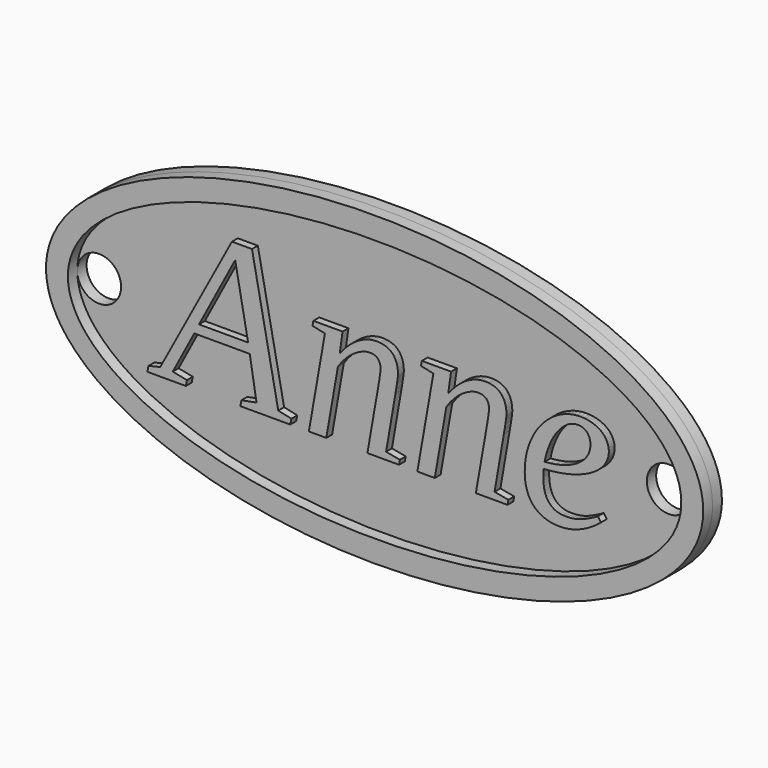
from build123d import *

# Parameters (mm, degrees)
F0_R     = 3
F1_DEPTH = 1.6
F2_DEPTH = 1.6
F3_DEPTH = 1


with BuildPart() as f1:
    # F0 (on Front) → F1 (new body)
    with BuildSketch(Plane.XZ):
        with BuildLine():
            add(Edge.make_bspline(
                [(45, 0), (45, 36.3730669589), (-22.5, 18.1865334795), (-90, 0), (-22.5, -18.1865334795), (45, -36.3730669589), (45, 0)],
                knots=[0, 0, 0, 2.0943951024, 2.0943951024, 4.1887902048, 4.1887902048, 6.2831853072, 6.2831853072, 6.2831853072], degree=2, weights=[1, 0.5, 1, 0.5, 1, 0.5, 1]))
        make_face()
        with BuildLine():
            add(Edge.make_bspline(
                [(42, 0), (42, 17.9999999333), (1.556e-07, 18), (-41.9999996887, 18.0000000667), (-42, 1.334e-07)],
                knots=[0, 0, 0, 1.5707963231, 1.5707963231, 3.1415926462, 3.1415926462, 3.1415926462], degree=2, weights=[1, 0.7071067825, 1, 0.7071067825, 1]))
            add(Edge.make_bspline(
                [(-42, 1.334e-07), (-42.0000003113, -17.9999999333), (-1.556e-07, -18), (42, -18.0000000667), (42, 0)],
                knots=[3.1415926462, 3.1415926462, 3.1415926462, 4.7123889767, 4.7123889767, 6.2831853072, 6.2831853072, 6.2831853072], degree=2, weights=[1, 0.7071067799, 1, 0.7071067799, 1]))
        make_face(mode=Mode.SUBTRACT)
        with BuildLine():
            add(Edge.make_bspline(
                [(-42, 1.334e-07), (-42.0000003113, -17.9999999333), (-1.556e-07, -18), (42, -18.0000000667), (42, 0)],
                knots=[3.1415926462, 3.1415926462, 3.1415926462, 4.7123889767, 4.7123889767, 6.2831853072, 6.2831853072, 6.2831853072], degree=2, weights=[1, 0.7071067799, 1, 0.7071067799, 1]))
            add(Edge.make_bspline(
                [(42, 0), (42, 17.9999999333), (1.556e-07, 18), (-41.9999996887, 18.0000000667), (-42, 1.334e-07)],
                knots=[0, 0, 0, 1.5707963231, 1.5707963231, 3.1415926462, 3.1415926462, 3.1415926462], degree=2, weights=[1, 0.7071067825, 1, 0.7071067825, 1]))
        make_face()
        Polygon((0.3302, 2.3205647869), (0.3306, 2.3652647869), (0.3252, 2.5233647869), (0.3185, 2.5995647869), (0.3091, 2.6737647869), (0.2969, 2.7461647869), (0.2821, 2.8165647869), (0.2645, 2.8851647869), (0.2443, 2.9517647869), (0.2214, 3.0164647869), (0.1957, 3.0792647869), (0.1674, 3.1401647869), (0.1363, 3.1991647869), (0.1026, 3.2561647869), (0.0662, 3.3113647869), (0.0271, 3.3645647869), (-0.0148, 3.4158647869), (-0.0595, 3.4646647869), (-0.1074, 3.5103647869), (-0.1585, 3.5528647869), (-0.2127, 3.5921647869), (-0.27, 3.6283647869), (-0.3305, 3.6614647869), (-0.3941, 3.6913647869), (-0.4609, 3.7181647869), (-0.5309, 3.7417647869), (-0.6039, 3.7621647869), (-0.6802, 3.7795647869), (-0.7596, 3.7936647869), (-0.8421, 3.8046647869), (-0.9278, 3.8125647869), (-1.0166, 3.8172647869), (-1.1086, 3.8188647869), (-1.2601, 3.8143647869), (-1.4126, 3.8008647869), (-1.566, 3.7783647869), (-1.7202, 3.7469647869), (-1.8754, 3.7064647869), (-2.0315, 3.6569647869), (-2.1884, 3.5984647869), (-2.3463, 3.5310647869), (-2.6602, 3.3835647869), (-2.9688, 3.2143647869), (-3.2719, 3.0237647869), (-3.5696, 2.8114647869), (-3.8593, 2.5802647869), (-4.1381, 2.3328647869), (-4.4062, 2.0693647869), (-4.6634, 1.7895647869), (-4.9054, 1.5089647869), (-5.1276, 1.2282647869), (-5.33, 0.9476647869), (-5.5126, 0.6669647869), (-7.0957, -8.4000352131), (-9.4848, -8.4000352131), (-7.2828, 4.1354647869), (-8.9811, 4.4952647869), (-8.8659, 5.1429647869), (-4.8649, 5.1429647869), (-5.2535, 2.3796647869), (-4.9774, 2.7241647869), (-4.4089, 3.3646647869), (-4.1165, 3.6605647869), (-3.8125, 3.9376647869), (-3.5049, 4.1930647869), (-3.1936, 4.4269647869), (-2.8788, 4.6392647869), (-2.5541, 4.8290647869), (-2.2276, 4.9954647869), (-1.8992, 5.1384647869), (-1.5691, 5.2580647869), (-1.23, 5.3588647869), (-0.8891, 5.4307647869), (-0.5464, 5.4739647869), (-0.2019, 5.4883647869), (0.1211, 5.4775647869), (0.2764, 5.4640647869), (0.4278, 5.4451647869), (0.5751, 5.4208647869), (0.7183, 5.3912647869), (0.8575, 5.3561647869), (0.9927, 5.3156647869), (1.1267, 5.2693647869), (1.2553, 5.2167647869), (1.3786, 5.1577647869), (1.4964, 5.0925647869), (1.6088, 5.0210647869), (1.7159, 4.9432647869), (1.8175, 4.8591647869), (1.9138, 4.7687647869), (2.008, 4.6720647869), (2.0964, 4.5690647869), (2.1789, 4.4597647869), (2.2556, 4.3441647869), (2.3264, 4.2222647869), (2.3914, 4.0941647869), (2.4506, 3.9596647869), (2.5039, 3.8188647869), (2.5545, 3.6715647869), (2.5983, 3.5175647869), (2.6354, 3.3567647869), (2.6658, 3.1892647869), (2.6894, 3.0149647869), (2.7062, 2.8339647869), (2.7164, 2.6461647869), (2.7197, 2.4516647869), (2.7196, 2.4295647869), (2.7191, 2.4064647869), (2.717, 2.3571647869), (2.7137, 2.3038647869), (2.7089, 2.2465647869), (2.7029, 2.1851647869), (2.6954, 2.1196647869), (2.6867, 2.0502647869), (2.6766, 1.9766647869), (2.6604, 1.8291647869), (2.6406, 1.6744647869), (2.6172, 1.5125647869), (2.5902, 1.3434647869), (2.5614, 1.1689647869), (2.5039, 0.8091647869), (2.4751, 0.6238647869), (2.4463, 0.4466647869), (2.3887, 0.1083647869), (2.3599, -0.0526352131), (1.0934, -7.4069352131), (2.9788, -7.7524352131), (2.8637, -8.4000352131), (-1.4684, -8.4000352131), (-0.0004, -0.0238352131), (0.0284, 0.1362647869), (0.086, 0.4673647869), (0.1148, 0.6382647869), (0.1426, 0.8100647869), (0.193, 1.1482647869), (0.2155, 1.3146647869), (0.2425, 1.4765647869), (0.2659, 1.6312647869), (0.2857, 1.7787647869), (0.3019, 1.9191647869), (0.3086, 1.9858647869), (0.3145, 2.0495647869), (0.3194, 2.1100647869), (0.3234, 2.1673647869), (0.3266, 2.2215647869), (0.3288, 2.2726647869), align=None, mode=Mode.SUBTRACT)
        Polygon((15.1836, 2.3205647869), (15.184, 2.3652647869), (15.1786, 2.5233647869), (15.1719, 2.5995647869), (15.1624, 2.6737647869), (15.1503, 2.7461647869), (15.1355, 2.8165647869), (15.1179, 2.8851647869), (15.0977, 2.9517647869), (15.0747, 3.0164647869), (15.0491, 3.0792647869), (15.0208, 3.1401647869), (14.9897, 3.1991647869), (14.956, 3.2561647869), (14.9196, 3.3113647869), (14.8805, 3.3645647869), (14.8386, 3.4158647869), (14.7939, 3.4646647869), (14.746, 3.5103647869), (14.6949, 3.5528647869), (14.6407, 3.5921647869), (14.5834, 3.6283647869), (14.5229, 3.6614647869), (14.4593, 3.6913647869), (14.3925, 3.7181647869), (14.3225, 3.7417647869), (14.2494, 3.7621647869), (14.1732, 3.7795647869), (14.0938, 3.7936647869), (14.0113, 3.8046647869), (13.9256, 3.8125647869), (13.8368, 3.8172647869), (13.7448, 3.8188647869), (13.5933, 3.8143647869), (13.4408, 3.8008647869), (13.2874, 3.7783647869), (13.1332, 3.7469647869), (12.978, 3.7064647869), (12.8219, 3.6569647869), (12.665, 3.5984647869), (12.5071, 3.5310647869), (12.1932, 3.3835647869), (11.8846, 3.2143647869), (11.5815, 3.0237647869), (11.2838, 2.8114647869), (10.9941, 2.5802647869), (10.7153, 2.3328647869), (10.4472, 2.0693647869), (10.19, 1.7895647869), (9.948, 1.5089647869), (9.7258, 1.2282647869), (9.5234, 0.9476647869), (9.3408, 0.6669647869), (7.7577, -8.4000352131), (5.3686, -8.4000352131), (7.5706, 4.1354647869), (5.8723, 4.4952647869), (5.9875, 5.1429647869), (9.9885, 5.1429647869), (9.5999, 2.3796647869), (9.876, 2.7241647869), (10.4445, 3.3646647869), (10.7369, 3.6605647869), (11.0409, 3.9376647869), (11.3485, 4.1930647869), (11.6598, 4.4269647869), (11.9746, 4.6392647869), (12.2993, 4.8290647869), (12.6258, 4.9954647869), (12.9542, 5.1384647869), (13.2843, 5.2580647869), (13.6234, 5.3588647869), (13.9643, 5.4307647869), (14.307, 5.4739647869), (14.6515, 5.4883647869), (14.9745, 5.4775647869), (15.1298, 5.4640647869), (15.2812, 5.4451647869), (15.4285, 5.4208647869), (15.5717, 5.3912647869), (15.7109, 5.3561647869), (15.8461, 5.3156647869), (15.9801, 5.2693647869), (16.1087, 5.2167647869), (16.232, 5.1577647869), (16.3498, 5.0925647869), (16.4622, 5.0210647869), (16.5693, 4.9432647869), (16.6709, 4.8591647869), (16.7672, 4.7687647869), (16.8614, 4.6720647869), (16.9498, 4.5690647869), (17.0323, 4.4597647869), (17.109, 4.3441647869), (17.1798, 4.2222647869), (17.2448, 4.0941647869), (17.304, 3.9596647869), (17.3572, 3.8188647869), (17.4078, 3.6715647869), (17.4517, 3.5175647869), (17.4888, 3.3567647869), (17.5192, 3.1892647869), (17.5428, 3.0149647869), (17.5596, 2.8339647869), (17.5698, 2.6461647869), (17.5731, 2.4516647869), (17.573, 2.4295647869), (17.5725, 2.4064647869), (17.5704, 2.3571647869), (17.5671, 2.3038647869), (17.5623, 2.2465647869), (17.5563, 2.1851647869), (17.5488, 2.1196647869), (17.5401, 2.0502647869), (17.53, 1.9766647869), (17.5138, 1.8291647869), (17.494, 1.6744647869), (17.4706, 1.5125647869), (17.4436, 1.3434647869), (17.4148, 1.1689647869), (17.3572, 0.8091647869), (17.3285, 0.6238647869), (17.2997, 0.4466647869), (17.2421, 0.1083647869), (17.2133, -0.0526352131), (15.9468, -7.4069352131), (17.8322, -7.7524352131), (17.7171, -8.4000352131), (13.385, -8.4000352131), (14.853, -0.0238352131), (14.8818, 0.1362647869), (14.9394, 0.4673647869), (14.9682, 0.6382647869), (14.996, 0.8100647869), (15.0464, 1.1482647869), (15.0689, 1.3146647869), (15.0959, 1.4765647869), (15.1193, 1.6312647869), (15.1391, 1.7787647869), (15.1553, 1.9191647869), (15.162, 1.9858647869), (15.1678, 2.0495647869), (15.1728, 2.1100647869), (15.1768, 2.1673647869), (15.18, 2.2215647869), (15.1822, 2.2726647869), align=None, mode=Mode.SUBTRACT)
        Polygon((31.5875, 2.6947647869), (31.5918, 2.5379647869), (31.5826, 2.3056647869), (31.5549, 2.0765647869), (31.5088, 1.8505647869), (31.4443, 1.6276647869), (31.3613, 1.4079647869), (31.2599, 1.1914647869), (31.14, 0.9779647869), (31.0017, 0.7677647869), (30.8456, 0.5615647869), (30.6725, 0.3602647869), (30.4822, 0.1639647869), (30.2749, -0.0274352131), (30.0505, -0.2138352131), (29.809, -0.3953352131), (29.5504, -0.5718352131), (29.2747, -0.7434352131), (28.9855, -0.9057352131), (28.6792, -1.0618352131), (28.3558, -1.2116352131), (28.0153, -1.3551352131), (27.6578, -1.4922352131), (27.2831, -1.6231352131), (26.4826, -1.8660352131), (25.6244, -2.0702352131), (24.7052, -2.2366352131), (23.7247, -2.3652352131), (22.6831, -2.4561352131), (22.6812, -2.4728352131), (22.6792, -2.4907352131), (22.6772, -2.5097352131), (22.675, -2.5298352131), (22.6727, -2.5511352131), (22.6702, -2.5734352131), (22.6677, -2.5969352131), (22.6651, -2.6216352131), (22.6594, -2.6742352131), (22.6534, -2.7313352131), (22.6469, -2.7929352131), (22.6399, -2.8590352131), (22.6365, -2.9290352131), (22.6311, -3.0783352131), (22.6275, -3.2402352131), (22.6257, -3.4147352131), (22.6255, -3.5067352131), (22.6336, -3.8566352131), (22.6579, -4.2011352131), (22.6983, -4.5402352131), (22.755, -4.8739352131), (22.7941, -5.0372352131), (22.8396, -5.1960352131), (22.8913, -5.3502352131), (22.9493, -5.5000352131), (23.0136, -5.6453352131), (23.0842, -5.7860352131), (23.1611, -5.9223352131), (23.2444, -6.0541352131), (23.3345, -6.1805352131), (23.4323, -6.3005352131), (23.5378, -6.4143352131), (23.6509, -6.5218352131), (23.7717, -6.6230352131), (23.9001, -6.7179352131), (24.0361, -6.8065352131), (24.1798, -6.8888352131), (24.3323, -6.9597352131), (24.4947, -7.0211352131), (24.6669, -7.0730352131), (24.8491, -7.1155352131), (25.0411, -7.1486352131), (25.2431, -7.1722352131), (25.4549, -7.1863352131), (25.6766, -7.1911352131), (25.9973, -7.1843352131), (26.3117, -7.1641352131), (26.6198, -7.1303352131), (26.9215, -7.0831352131), (27.217, -7.0224352131), (27.5062, -6.9482352131), (27.7891, -6.8605352131), (28.0657, -6.7593352131), (28.6036, -6.5290352131), (29.6255, -6.0253352131), (30.1094, -5.7518352131), (30.5268, -6.3563352131), (30.2866, -6.5524352131), (30.0266, -6.7521352131), (29.7469, -6.9554352131), (29.4474, -7.1623352131), (29.1307, -7.3665352131), (28.7997, -7.5617352131), (28.0945, -7.9251352131), (27.7293, -8.0834352131), (27.3533, -8.2273352131), (26.9665, -8.3568352131), (26.5689, -8.4720352131), (26.1642, -8.5664352131), (25.7558, -8.6339352131), (25.3438, -8.6743352131), (24.9282, -8.6878352131), (24.6273, -8.6824352131), (24.3364, -8.6663352131), (24.0553, -8.6393352131), (23.7841, -8.6015352131), (23.5227, -8.5529352131), (23.2713, -8.4935352131), (23.0298, -8.4234352131), (22.7982, -8.3424352131), (22.5762, -8.2480352131), (22.3637, -8.1445352131), (22.1607, -8.0321352131), (21.967, -7.9107352131), (21.7829, -7.7802352131), (21.6081, -7.6408352131), (21.4429, -7.4924352131), (21.287, -7.3350352131), (21.1406, -7.1686352131), (21.0037, -6.9932352131), (20.8762, -6.8088352131), (20.7581, -6.6154352131), (20.6495, -6.4130352131), (20.5503, -6.2016352131), (20.4606, -5.9812352131), (20.3803, -5.7518352131), (20.3095, -5.5144352131), (20.2481, -5.2697352131), (20.1961, -5.0179352131), (20.1536, -4.7588352131), (20.1206, -4.4925352131), (20.0828, -3.9384352131), (20.0781, -3.6506352131), (20.0961, -3.0173352131), (20.15, -2.3985352131), (20.24, -1.7940352131), (20.3659, -1.2039352131), (20.5242, -0.6247352131), (20.7113, -0.0670352131), (20.9272, 0.4690647869), (21.1719, 0.9836647869), (21.4435, 1.4819647869), (21.7404, 1.9550647869), (22.0624, 2.4030647869), (22.4096, 2.8258647869), (22.7766, 3.2278647869), (23.158, 3.5993647869), (23.5538, 3.9403647869), (23.964, 4.2506647869), (24.3939, 4.5285647869), (24.8347, 4.7723647869), (25.2862, 4.9819647869), (25.7486, 5.1573647869), (26.2253, 5.3021647869), (26.7057, 5.4055647869), (27.1896, 5.4676647869), (27.6771, 5.4883647869), (28.1251, 5.4739647869), (28.3396, 5.4559647869), (28.5478, 5.4307647869), (28.7498, 5.3984647869), (28.9454, 5.3588647869), (29.1348, 5.3120647869), (29.3178, 5.2580647869), (29.4977, 5.2011647869), (29.6704, 5.1384647869), (29.8359, 5.0698647869), (29.9943, 4.9954647869), (30.1454, 4.9151647869), (30.2893, 4.8290647869), (30.426, 4.7370647869), (30.5556, 4.6392647869), (30.6777, 4.5395647869), (30.7921, 4.4350647869), (30.8989, 4.3255647869), (30.9981, 4.2110647869), (31.0896, 4.0916647869), (31.1735, 3.9672647869), (31.2497, 3.8379647869), (31.3183, 3.7037647869), (31.3824, 3.5690647869), (31.438, 3.4311647869), (31.485, 3.2901647869), (31.5234, 3.1460647869), (31.5533, 2.9987647869), (31.5747, 2.8482647869), align=None, mode=Mode.SUBTRACT)
        with BuildLine():
            ThreePointArc((-36, 0), (-39.0000000667, -3), (-42, 1.334e-07))
            ThreePointArc((-42, 1.334e-07), (-38.9999999333, 3), (-36, 0))
        make_face(mode=Mode.SUBTRACT)
        Polygon((-28.1233, -7.2486352131), (-26.1804, -7.6372352131), (-26.3243, -8.4000352131), (-31.5918, -8.4000352131), (-31.4479, -7.6372352131), (-29.836, -7.2486352131), (-20.0205, 11.0581647869), (-17.2716, 11.0581647869), (-13.6736, -7.2486352131), (-11.8746, -7.6372352131), (-12.0329, -8.4000352131), (-18.8692, -8.4000352131), (-18.7109, -7.6372352131), (-16.6528, -7.2486352131), (-17.5739, -1.6789352131), (-25.1729, -1.6789352131), align=None, mode=Mode.SUBTRACT)
        with Locations((39, 0)):
            Circle(F0_R, mode=Mode.SUBTRACT)
        Polygon((-26.3243, -8.4000352131), (-26.1804, -7.6372352131), (-28.1233, -7.2486352131), (-25.1729, -1.6789352131), (-17.5739, -1.6789352131), (-16.6528, -7.2486352131), (-18.7109, -7.6372352131), (-18.8692, -8.4000352131), (-12.0329, -8.4000352131), (-11.8746, -7.6372352131), (-13.6736, -7.2486352131), (-17.2716, 11.0581647869), (-20.0205, 11.0581647869), (-29.836, -7.2486352131), (-31.4479, -7.6372352131), (-31.5918, -8.4000352131), align=None)
        Polygon((-24.5253, -0.3836352131), (-19.5744, 8.9856647869), (-17.8042, -0.3836352131), align=None, mode=Mode.SUBTRACT)
        Polygon((31.5826, 2.3056647869), (31.5918, 2.5379647869), (31.5875, 2.6947647869), (31.5747, 2.8482647869), (31.5533, 2.9987647869), (31.5234, 3.1460647869), (31.485, 3.2901647869), (31.438, 3.4311647869), (31.3824, 3.5690647869), (31.3183, 3.7037647869), (31.2497, 3.8379647869), (31.1735, 3.9672647869), (31.0896, 4.0916647869), (30.9981, 4.2110647869), (30.8989, 4.3255647869), (30.7921, 4.4350647869), (30.6777, 4.5395647869), (30.5556, 4.6392647869), (30.426, 4.7370647869), (30.2893, 4.8290647869), (30.1454, 4.9151647869), (29.9943, 4.9954647869), (29.8359, 5.0698647869), (29.6704, 5.1384647869), (29.4977, 5.2011647869), (29.3178, 5.2580647869), (29.1348, 5.3120647869), (28.9454, 5.3588647869), (28.7498, 5.3984647869), (28.5478, 5.4307647869), (28.3396, 5.4559647869), (28.1251, 5.4739647869), (27.6771, 5.4883647869), (27.1896, 5.4676647869), (26.7057, 5.4055647869), (26.2253, 5.3021647869), (25.7486, 5.1573647869), (25.2862, 4.9819647869), (24.8347, 4.7723647869), (24.3939, 4.5285647869), (23.964, 4.2506647869), (23.5538, 3.9403647869), (23.158, 3.5993647869), (22.7766, 3.2278647869), (22.4096, 2.8258647869), (22.0624, 2.4030647869), (21.7404, 1.9550647869), (21.4435, 1.4819647869), (21.1719, 0.9836647869), (20.9272, 0.4690647869), (20.7113, -0.0670352131), (20.5242, -0.6247352131), (20.3659, -1.2039352131), (20.24, -1.7940352131), (20.15, -2.3985352131), (20.0961, -3.0173352131), (20.0781, -3.6506352131), (20.0828, -3.9384352131), (20.1206, -4.4925352131), (20.1536, -4.7588352131), (20.1961, -5.0179352131), (20.2481, -5.2697352131), (20.3095, -5.5144352131), (20.3803, -5.7518352131), (20.4606, -5.9812352131), (20.5503, -6.2016352131), (20.6495, -6.4130352131), (20.7581, -6.6154352131), (20.8762, -6.8088352131), (21.0037, -6.9932352131), (21.1406, -7.1686352131), (21.287, -7.3350352131), (21.4429, -7.4924352131), (21.6081, -7.6408352131), (21.7829, -7.7802352131), (21.967, -7.9107352131), (22.1607, -8.0321352131), (22.3637, -8.1445352131), (22.5762, -8.2480352131), (22.7982, -8.3424352131), (23.0298, -8.4234352131), (23.2713, -8.4935352131), (23.5227, -8.5529352131), (23.7841, -8.6015352131), (24.0553, -8.6393352131), (24.3364, -8.6663352131), (24.6273, -8.6824352131), (24.9282, -8.6878352131), (25.3438, -8.6743352131), (25.7558, -8.6339352131), (26.1642, -8.5664352131), (26.5689, -8.4720352131), (26.9665, -8.3568352131), (27.3533, -8.2273352131), (27.7293, -8.0834352131), (28.0945, -7.9251352131), (28.7997, -7.5617352131), (29.1307, -7.3665352131), (29.4474, -7.1623352131), (29.7469, -6.9554352131), (30.0266, -6.7521352131), (30.2866, -6.5524352131), (30.5268, -6.3563352131), (30.1094, -5.7518352131), (29.6255, -6.0253352131), (28.6036, -6.5290352131), (28.0657, -6.7593352131), (27.7891, -6.8605352131), (27.5062, -6.9482352131), (27.217, -7.0224352131), (26.9215, -7.0831352131), (26.6198, -7.1303352131), (26.3117, -7.1641352131), (25.9973, -7.1843352131), (25.6766, -7.1911352131), (25.4549, -7.1863352131), (25.2431, -7.1722352131), (25.0411, -7.1486352131), (24.8491, -7.1155352131), (24.6669, -7.0730352131), (24.4947, -7.0211352131), (24.3323, -6.9597352131), (24.1798, -6.8888352131), (24.0361, -6.8065352131), (23.9001, -6.7179352131), (23.7717, -6.6230352131), (23.6509, -6.5218352131), (23.5378, -6.4143352131), (23.4323, -6.3005352131), (23.3345, -6.1805352131), (23.2444, -6.0541352131), (23.1611, -5.9223352131), (23.0842, -5.7860352131), (23.0136, -5.6453352131), (22.9493, -5.5000352131), (22.8913, -5.3502352131), (22.8396, -5.1960352131), (22.7941, -5.0372352131), (22.755, -4.8739352131), (22.6983, -4.5402352131), (22.6579, -4.2011352131), (22.6336, -3.8566352131), (22.6255, -3.5067352131), (22.6257, -3.4147352131), (22.6275, -3.2402352131), (22.6311, -3.0783352131), (22.6365, -2.9290352131), (22.6399, -2.8590352131), (22.6469, -2.7929352131), (22.6534, -2.7313352131), (22.6594, -2.6742352131), (22.6651, -2.6216352131), (22.6677, -2.5969352131), (22.6702, -2.5734352131), (22.6727, -2.5511352131), (22.675, -2.5298352131), (22.6772, -2.5097352131), (22.6792, -2.4907352131), (22.6812, -2.4728352131), (22.6831, -2.4561352131), (23.7247, -2.3652352131), (24.7052, -2.2366352131), (25.6244, -2.0702352131), (26.4826, -1.8660352131), (27.2831, -1.6231352131), (27.6578, -1.4922352131), (28.0153, -1.3551352131), (28.3558, -1.2116352131), (28.6792, -1.0618352131), (28.9855, -0.9057352131), (29.2747, -0.7434352131), (29.5504, -0.5718352131), (29.809, -0.3953352131), (30.0505, -0.2138352131), (30.2749, -0.0274352131), (30.4822, 0.1639647869), (30.6725, 0.3602647869), (30.8456, 0.5615647869), (31.0017, 0.7677647869), (31.14, 0.9779647869), (31.2599, 1.1914647869), (31.3613, 1.4079647869), (31.4443, 1.6276647869), (31.5088, 1.8505647869), (31.5549, 2.0765647869), align=None)
        Polygon((23.5583, -1.4756352131), (22.7982, -1.5493352131), (22.9061, -1.0303352131), (23.0429, -0.5095352131), (23.2084, 0.0130647869), (23.4027, 0.5374647869), (23.6221, 1.0564647869), (23.8632, 1.5485647869), (24.1259, 2.0135647869), (24.4101, 2.4516647869), (24.5635, 2.6589647869), (24.8837, 3.0439647869), (25.0506, 3.2215647869), (25.2219, 3.3893647869), (25.3978, 3.5472647869), (25.5781, 3.6951647869), (25.763, 3.8332647869), (25.9516, 3.9614647869), (26.1435, 4.0725647869), (26.3384, 4.1665647869), (26.5366, 4.2434647869), (26.7378, 4.3032647869), (26.9422, 4.3459647869), (27.1498, 4.3716647869), (27.3605, 4.3801647869), (27.4633, 4.3781647869), (27.5629, 4.3720647869), (27.6594, 4.3619647869), (27.7527, 4.3477647869), (27.8429, 4.3295647869), (27.9299, 4.3073647869), (28.0138, 4.2809647869), (28.0945, 4.2506647869), (28.1721, 4.2162647869), (28.2465, 4.1777647869), (28.3178, 4.1352647869), (28.3859, 4.0887647869), (28.4509, 4.0381647869), (28.5128, 3.9834647869), (28.5715, 3.9247647869), (28.627, 3.8620647869), (28.681, 3.7961647869), (28.7316, 3.7280647869), (28.7786, 3.6576647869), (28.8222, 3.5849647869), (28.8623, 3.5101647869), (28.8989, 3.4329647869), (28.932, 3.3535647869), (28.9616, 3.2719647869), (28.9878, 3.1880647869), (29.0104, 3.1019647869), (29.0296, 3.0135647869), (29.0453, 2.9229647869), (29.0575, 2.8300647869), (29.0662, 2.7349647869), (29.0732, 2.5379647869), (29.0671, 2.3551647869), (29.0489, 2.1736647869), (29.0185, 1.9935647869), (28.976, 1.8147647869), (28.9214, 1.6373647869), (28.8546, 1.4612647869), (28.7757, 1.2865647869), (28.6846, 1.1131647869), (28.5811, 0.9458647869), (28.4651, 0.7821647869), (28.3365, 0.6220647869), (28.1952, 0.4655647869), (28.0414, 0.3125647869), (27.875, 0.1632647869), (27.696, 0.0175647869), (27.5044, -0.1245352131), (27.3038, -0.2588352131), (27.0906, -0.3881352131), (26.8649, -0.5124352131), (26.6265, -0.6318352131), (26.3755, -0.7463352131), (26.112, -0.8558352131), (25.8358, -0.9604352131), (25.5471, -1.0600352131), (25.246, -1.1495352131), (24.9327, -1.2309352131), (24.2698, -1.3694352131), align=None, mode=Mode.SUBTRACT)
        Polygon((0.3252, 2.5233647869), (0.3306, 2.3652647869), (0.3302, 2.3205647869), (0.3288, 2.2726647869), (0.3266, 2.2215647869), (0.3234, 2.1673647869), (0.3194, 2.1100647869), (0.3145, 2.0495647869), (0.3086, 1.9858647869), (0.3019, 1.9191647869), (0.2857, 1.7787647869), (0.2659, 1.6312647869), (0.2425, 1.4765647869), (0.2155, 1.3146647869), (0.193, 1.1482647869), (0.1426, 0.8100647869), (0.1148, 0.6382647869), (0.086, 0.4673647869), (0.0284, 0.1362647869), (-0.0004, -0.0238352131), (-1.4684, -8.4000352131), (2.8637, -8.4000352131), (2.9788, -7.7524352131), (1.0934, -7.4069352131), (2.3599, -0.0526352131), (2.3887, 0.1083647869), (2.4463, 0.4466647869), (2.4751, 0.6238647869), (2.5039, 0.8091647869), (2.5614, 1.1689647869), (2.5902, 1.3434647869), (2.6172, 1.5125647869), (2.6406, 1.6744647869), (2.6604, 1.8291647869), (2.6766, 1.9766647869), (2.6867, 2.0502647869), (2.6954, 2.1196647869), (2.7029, 2.1851647869), (2.7089, 2.2465647869), (2.7137, 2.3038647869), (2.717, 2.3571647869), (2.7191, 2.4064647869), (2.7196, 2.4295647869), (2.7197, 2.4516647869), (2.7164, 2.6461647869), (2.7062, 2.8339647869), (2.6894, 3.0149647869), (2.6658, 3.1892647869), (2.6354, 3.3567647869), (2.5983, 3.5175647869), (2.5545, 3.6715647869), (2.5039, 3.8188647869), (2.4506, 3.9596647869), (2.3914, 4.0941647869), (2.3264, 4.2222647869), (2.2556, 4.3441647869), (2.1789, 4.4597647869), (2.0964, 4.5690647869), (2.008, 4.6720647869), (1.9138, 4.7687647869), (1.8175, 4.8591647869), (1.7159, 4.9432647869), (1.6088, 5.0210647869), (1.4964, 5.0925647869), (1.3786, 5.1577647869), (1.2553, 5.2167647869), (1.1267, 5.2693647869), (0.9927, 5.3156647869), (0.8575, 5.3561647869), (0.7183, 5.3912647869), (0.5751, 5.4208647869), (0.4278, 5.4451647869), (0.2764, 5.4640647869), (0.1211, 5.4775647869), (-0.2019, 5.4883647869), (-0.5464, 5.4739647869), (-0.8891, 5.4307647869), (-1.23, 5.3588647869), (-1.5691, 5.2580647869), (-1.8992, 5.1384647869), (-2.2276, 4.9954647869), (-2.5541, 4.8290647869), (-2.8788, 4.6392647869), (-3.1936, 4.4269647869), (-3.5049, 4.1930647869), (-3.8125, 3.9376647869), (-4.1165, 3.6605647869), (-4.4089, 3.3646647869), (-4.9774, 2.7241647869), (-5.2535, 2.3796647869), (-4.8649, 5.1429647869), (-8.8659, 5.1429647869), (-8.9811, 4.4952647869), (-7.2828, 4.1354647869), (-9.4848, -8.4000352131), (-7.0957, -8.4000352131), (-5.5126, 0.6669647869), (-5.33, 0.9476647869), (-5.1276, 1.2282647869), (-4.9054, 1.5089647869), (-4.6634, 1.7895647869), (-4.4062, 2.0693647869), (-4.1381, 2.3328647869), (-3.8593, 2.5802647869), (-3.5696, 2.8114647869), (-3.2719, 3.0237647869), (-2.9688, 3.2143647869), (-2.6602, 3.3835647869), (-2.3463, 3.5310647869), (-2.1884, 3.5984647869), (-2.0315, 3.6569647869), (-1.8754, 3.7064647869), (-1.7202, 3.7469647869), (-1.566, 3.7783647869), (-1.4126, 3.8008647869), (-1.2601, 3.8143647869), (-1.1086, 3.8188647869), (-1.0166, 3.8172647869), (-0.9278, 3.8125647869), (-0.8421, 3.8046647869), (-0.7596, 3.7936647869), (-0.6802, 3.7795647869), (-0.6039, 3.7621647869), (-0.5309, 3.7417647869), (-0.4609, 3.7181647869), (-0.3941, 3.6913647869), (-0.3305, 3.6614647869), (-0.27, 3.6283647869), (-0.2127, 3.5921647869), (-0.1585, 3.5528647869), (-0.1074, 3.5103647869), (-0.0595, 3.4646647869), (-0.0148, 3.4158647869), (0.0271, 3.3645647869), (0.0662, 3.3113647869), (0.1026, 3.2561647869), (0.1363, 3.1991647869), (0.1674, 3.1401647869), (0.1957, 3.0792647869), (0.2214, 3.0164647869), (0.2443, 2.9517647869), (0.2645, 2.8851647869), (0.2821, 2.8165647869), (0.2969, 2.7461647869), (0.3091, 2.6737647869), (0.3185, 2.5995647869), align=None)
        Polygon((15.1786, 2.5233647869), (15.184, 2.3652647869), (15.1836, 2.3205647869), (15.1822, 2.2726647869), (15.18, 2.2215647869), (15.1768, 2.1673647869), (15.1728, 2.1100647869), (15.1678, 2.0495647869), (15.162, 1.9858647869), (15.1553, 1.9191647869), (15.1391, 1.7787647869), (15.1193, 1.6312647869), (15.0959, 1.4765647869), (15.0689, 1.3146647869), (15.0464, 1.1482647869), (14.996, 0.8100647869), (14.9682, 0.6382647869), (14.9394, 0.4673647869), (14.8818, 0.1362647869), (14.853, -0.0238352131), (13.385, -8.4000352131), (17.7171, -8.4000352131), (17.8322, -7.7524352131), (15.9468, -7.4069352131), (17.2133, -0.0526352131), (17.2421, 0.1083647869), (17.2997, 0.4466647869), (17.3285, 0.6238647869), (17.3572, 0.8091647869), (17.4148, 1.1689647869), (17.4436, 1.3434647869), (17.4706, 1.5125647869), (17.494, 1.6744647869), (17.5138, 1.8291647869), (17.53, 1.9766647869), (17.5401, 2.0502647869), (17.5488, 2.1196647869), (17.5563, 2.1851647869), (17.5623, 2.2465647869), (17.5671, 2.3038647869), (17.5704, 2.3571647869), (17.5725, 2.4064647869), (17.573, 2.4295647869), (17.5731, 2.4516647869), (17.5698, 2.6461647869), (17.5596, 2.8339647869), (17.5428, 3.0149647869), (17.5192, 3.1892647869), (17.4888, 3.3567647869), (17.4517, 3.5175647869), (17.4078, 3.6715647869), (17.3572, 3.8188647869), (17.304, 3.9596647869), (17.2448, 4.0941647869), (17.1798, 4.2222647869), (17.109, 4.3441647869), (17.0323, 4.4597647869), (16.9498, 4.5690647869), (16.8614, 4.6720647869), (16.7672, 4.7687647869), (16.6709, 4.8591647869), (16.5693, 4.9432647869), (16.4622, 5.0210647869), (16.3498, 5.0925647869), (16.232, 5.1577647869), (16.1087, 5.2167647869), (15.9801, 5.2693647869), (15.8461, 5.3156647869), (15.7109, 5.3561647869), (15.5717, 5.3912647869), (15.4285, 5.4208647869), (15.2812, 5.4451647869), (15.1298, 5.4640647869), (14.9745, 5.4775647869), (14.6515, 5.4883647869), (14.307, 5.4739647869), (13.9643, 5.4307647869), (13.6234, 5.3588647869), (13.2843, 5.2580647869), (12.9542, 5.1384647869), (12.6258, 4.9954647869), (12.2993, 4.8290647869), (11.9746, 4.6392647869), (11.6598, 4.4269647869), (11.3485, 4.1930647869), (11.0409, 3.9376647869), (10.7369, 3.6605647869), (10.4445, 3.3646647869), (9.876, 2.7241647869), (9.5999, 2.3796647869), (9.9885, 5.1429647869), (5.9875, 5.1429647869), (5.8723, 4.4952647869), (7.5706, 4.1354647869), (5.3686, -8.4000352131), (7.7577, -8.4000352131), (9.3408, 0.6669647869), (9.5234, 0.9476647869), (9.7258, 1.2282647869), (9.948, 1.5089647869), (10.19, 1.7895647869), (10.4472, 2.0693647869), (10.7153, 2.3328647869), (10.9941, 2.5802647869), (11.2838, 2.8114647869), (11.5815, 3.0237647869), (11.8846, 3.2143647869), (12.1932, 3.3835647869), (12.5071, 3.5310647869), (12.665, 3.5984647869), (12.8219, 3.6569647869), (12.978, 3.7064647869), (13.1332, 3.7469647869), (13.2874, 3.7783647869), (13.4408, 3.8008647869), (13.5933, 3.8143647869), (13.7448, 3.8188647869), (13.8368, 3.8172647869), (13.9256, 3.8125647869), (14.0113, 3.8046647869), (14.0938, 3.7936647869), (14.1732, 3.7795647869), (14.2494, 3.7621647869), (14.3225, 3.7417647869), (14.3925, 3.7181647869), (14.4593, 3.6913647869), (14.5229, 3.6614647869), (14.5834, 3.6283647869), (14.6407, 3.5921647869), (14.6949, 3.5528647869), (14.746, 3.5103647869), (14.7939, 3.4646647869), (14.8386, 3.4158647869), (14.8805, 3.3645647869), (14.9196, 3.3113647869), (14.956, 3.2561647869), (14.9897, 3.1991647869), (15.0208, 3.1401647869), (15.0491, 3.0792647869), (15.0747, 3.0164647869), (15.0977, 2.9517647869), (15.1179, 2.8851647869), (15.1355, 2.8165647869), (15.1503, 2.7461647869), (15.1624, 2.6737647869), (15.1719, 2.5995647869), align=None)
        Polygon((-17.8042, -0.3836352131), (-19.5744, 8.9856647869), (-24.5253, -0.3836352131), align=None)
        Polygon((22.9061, -1.0303352131), (22.7982, -1.5493352131), (23.5583, -1.4756352131), (24.2698, -1.3694352131), (24.9327, -1.2309352131), (25.246, -1.1495352131), (25.5471, -1.0600352131), (25.8358, -0.9604352131), (26.112, -0.8558352131), (26.3755, -0.7463352131), (26.6265, -0.6318352131), (26.8649, -0.5124352131), (27.0906, -0.3881352131), (27.3038, -0.2588352131), (27.5044, -0.1245352131), (27.696, 0.0175647869), (27.875, 0.1632647869), (28.0414, 0.3125647869), (28.1952, 0.4655647869), (28.3365, 0.6220647869), (28.4651, 0.7821647869), (28.5811, 0.9458647869), (28.6846, 1.1131647869), (28.7757, 1.2865647869), (28.8546, 1.4612647869), (28.9214, 1.6373647869), (28.976, 1.8147647869), (29.0185, 1.9935647869), (29.0489, 2.1736647869), (29.0671, 2.3551647869), (29.0732, 2.5379647869), (29.0662, 2.7349647869), (29.0575, 2.8300647869), (29.0453, 2.9229647869), (29.0296, 3.0135647869), (29.0104, 3.1019647869), (28.9878, 3.1880647869), (28.9616, 3.2719647869), (28.932, 3.3535647869), (28.8989, 3.4329647869), (28.8623, 3.5101647869), (28.8222, 3.5849647869), (28.7786, 3.6576647869), (28.7316, 3.7280647869), (28.681, 3.7961647869), (28.627, 3.8620647869), (28.5715, 3.9247647869), (28.5128, 3.9834647869), (28.4509, 4.0381647869), (28.3859, 4.0887647869), (28.3178, 4.1352647869), (28.2465, 4.1777647869), (28.1721, 4.2162647869), (28.0945, 4.2506647869), (28.0138, 4.2809647869), (27.9299, 4.3073647869), (27.8429, 4.3295647869), (27.7527, 4.3477647869), (27.6594, 4.3619647869), (27.5629, 4.3720647869), (27.4633, 4.3781647869), (27.3605, 4.3801647869), (27.1498, 4.3716647869), (26.9422, 4.3459647869), (26.7378, 4.3032647869), (26.5366, 4.2434647869), (26.3384, 4.1665647869), (26.1435, 4.0725647869), (25.9516, 3.9614647869), (25.763, 3.8332647869), (25.5781, 3.6951647869), (25.3978, 3.5472647869), (25.2219, 3.3893647869), (25.0506, 3.2215647869), (24.8837, 3.0439647869), (24.5635, 2.6589647869), (24.4101, 2.4516647869), (24.1259, 2.0135647869), (23.8632, 1.5485647869), (23.6221, 1.0564647869), (23.4027, 0.5374647869), (23.2084, 0.0130647869), (23.0429, -0.5095352131), align=None)
    extrude(amount=-F1_DEPTH)

    # F0 (on Front) → F2 (join)
    with BuildSketch(Plane.XZ):
        with BuildLine():
            add(Edge.make_bspline(
                [(45, 0), (45, 36.3730669589), (-22.5, 18.1865334795), (-90, 0), (-22.5, -18.1865334795), (45, -36.3730669589), (45, 0)],
                knots=[0, 0, 0, 2.0943951024, 2.0943951024, 4.1887902048, 4.1887902048, 6.2831853072, 6.2831853072, 6.2831853072], degree=2, weights=[1, 0.5, 1, 0.5, 1, 0.5, 1]))
        make_face()
        with BuildLine():
            add(Edge.make_bspline(
                [(42, 0), (42, 17.9999999333), (1.556e-07, 18), (-41.9999996887, 18.0000000667), (-42, 1.334e-07)],
                knots=[0, 0, 0, 1.5707963231, 1.5707963231, 3.1415926462, 3.1415926462, 3.1415926462], degree=2, weights=[1, 0.7071067825, 1, 0.7071067825, 1]))
            add(Edge.make_bspline(
                [(-42, 1.334e-07), (-42.0000003113, -17.9999999333), (-1.556e-07, -18), (42, -18.0000000667), (42, 0)],
                knots=[3.1415926462, 3.1415926462, 3.1415926462, 4.7123889767, 4.7123889767, 6.2831853072, 6.2831853072, 6.2831853072], degree=2, weights=[1, 0.7071067799, 1, 0.7071067799, 1]))
        make_face(mode=Mode.SUBTRACT)
    extrude(amount=F2_DEPTH)

    # F0 (on Front) → F3 (join)
    with BuildSketch(Plane.XZ):
        Polygon((-26.3243, -8.4000352131), (-26.1804, -7.6372352131), (-28.1233, -7.2486352131), (-25.1729, -1.6789352131), (-17.5739, -1.6789352131), (-16.6528, -7.2486352131), (-18.7109, -7.6372352131), (-18.8692, -8.4000352131), (-12.0329, -8.4000352131), (-11.8746, -7.6372352131), (-13.6736, -7.2486352131), (-17.2716, 11.0581647869), (-20.0205, 11.0581647869), (-29.836, -7.2486352131), (-31.4479, -7.6372352131), (-31.5918, -8.4000352131), align=None)
        Polygon((-24.5253, -0.3836352131), (-19.5744, 8.9856647869), (-17.8042, -0.3836352131), align=None, mode=Mode.SUBTRACT)
        Polygon((0.3252, 2.5233647869), (0.3306, 2.3652647869), (0.3302, 2.3205647869), (0.3288, 2.2726647869), (0.3266, 2.2215647869), (0.3234, 2.1673647869), (0.3194, 2.1100647869), (0.3145, 2.0495647869), (0.3086, 1.9858647869), (0.3019, 1.9191647869), (0.2857, 1.7787647869), (0.2659, 1.6312647869), (0.2425, 1.4765647869), (0.2155, 1.3146647869), (0.193, 1.1482647869), (0.1426, 0.8100647869), (0.1148, 0.6382647869), (0.086, 0.4673647869), (0.0284, 0.1362647869), (-0.0004, -0.0238352131), (-1.4684, -8.4000352131), (2.8637, -8.4000352131), (2.9788, -7.7524352131), (1.0934, -7.4069352131), (2.3599, -0.0526352131), (2.3887, 0.1083647869), (2.4463, 0.4466647869), (2.4751, 0.6238647869), (2.5039, 0.8091647869), (2.5614, 1.1689647869), (2.5902, 1.3434647869), (2.6172, 1.5125647869), (2.6406, 1.6744647869), (2.6604, 1.8291647869), (2.6766, 1.9766647869), (2.6867, 2.0502647869), (2.6954, 2.1196647869), (2.7029, 2.1851647869), (2.7089, 2.2465647869), (2.7137, 2.3038647869), (2.717, 2.3571647869), (2.7191, 2.4064647869), (2.7196, 2.4295647869), (2.7197, 2.4516647869), (2.7164, 2.6461647869), (2.7062, 2.8339647869), (2.6894, 3.0149647869), (2.6658, 3.1892647869), (2.6354, 3.3567647869), (2.5983, 3.5175647869), (2.5545, 3.6715647869), (2.5039, 3.8188647869), (2.4506, 3.9596647869), (2.3914, 4.0941647869), (2.3264, 4.2222647869), (2.2556, 4.3441647869), (2.1789, 4.4597647869), (2.0964, 4.5690647869), (2.008, 4.6720647869), (1.9138, 4.7687647869), (1.8175, 4.8591647869), (1.7159, 4.9432647869), (1.6088, 5.0210647869), (1.4964, 5.0925647869), (1.3786, 5.1577647869), (1.2553, 5.2167647869), (1.1267, 5.2693647869), (0.9927, 5.3156647869), (0.8575, 5.3561647869), (0.7183, 5.3912647869), (0.5751, 5.4208647869), (0.4278, 5.4451647869), (0.2764, 5.4640647869), (0.1211, 5.4775647869), (-0.2019, 5.4883647869), (-0.5464, 5.4739647869), (-0.8891, 5.4307647869), (-1.23, 5.3588647869), (-1.5691, 5.2580647869), (-1.8992, 5.1384647869), (-2.2276, 4.9954647869), (-2.5541, 4.8290647869), (-2.8788, 4.6392647869), (-3.1936, 4.4269647869), (-3.5049, 4.1930647869), (-3.8125, 3.9376647869), (-4.1165, 3.6605647869), (-4.4089, 3.3646647869), (-4.9774, 2.7241647869), (-5.2535, 2.3796647869), (-4.8649, 5.1429647869), (-8.8659, 5.1429647869), (-8.9811, 4.4952647869), (-7.2828, 4.1354647869), (-9.4848, -8.4000352131), (-7.0957, -8.4000352131), (-5.5126, 0.6669647869), (-5.33, 0.9476647869), (-5.1276, 1.2282647869), (-4.9054, 1.5089647869), (-4.6634, 1.7895647869), (-4.4062, 2.0693647869), (-4.1381, 2.3328647869), (-3.8593, 2.5802647869), (-3.5696, 2.8114647869), (-3.2719, 3.0237647869), (-2.9688, 3.2143647869), (-2.6602, 3.3835647869), (-2.3463, 3.5310647869), (-2.1884, 3.5984647869), (-2.0315, 3.6569647869), (-1.8754, 3.7064647869), (-1.7202, 3.7469647869), (-1.566, 3.7783647869), (-1.4126, 3.8008647869), (-1.2601, 3.8143647869), (-1.1086, 3.8188647869), (-1.0166, 3.8172647869), (-0.9278, 3.8125647869), (-0.8421, 3.8046647869), (-0.7596, 3.7936647869), (-0.6802, 3.7795647869), (-0.6039, 3.7621647869), (-0.5309, 3.7417647869), (-0.4609, 3.7181647869), (-0.3941, 3.6913647869), (-0.3305, 3.6614647869), (-0.27, 3.6283647869), (-0.2127, 3.5921647869), (-0.1585, 3.5528647869), (-0.1074, 3.5103647869), (-0.0595, 3.4646647869), (-0.0148, 3.4158647869), (0.0271, 3.3645647869), (0.0662, 3.3113647869), (0.1026, 3.2561647869), (0.1363, 3.1991647869), (0.1674, 3.1401647869), (0.1957, 3.0792647869), (0.2214, 3.0164647869), (0.2443, 2.9517647869), (0.2645, 2.8851647869), (0.2821, 2.8165647869), (0.2969, 2.7461647869), (0.3091, 2.6737647869), (0.3185, 2.5995647869), align=None)
        Polygon((15.1786, 2.5233647869), (15.184, 2.3652647869), (15.1836, 2.3205647869), (15.1822, 2.2726647869), (15.18, 2.2215647869), (15.1768, 2.1673647869), (15.1728, 2.1100647869), (15.1678, 2.0495647869), (15.162, 1.9858647869), (15.1553, 1.9191647869), (15.1391, 1.7787647869), (15.1193, 1.6312647869), (15.0959, 1.4765647869), (15.0689, 1.3146647869), (15.0464, 1.1482647869), (14.996, 0.8100647869), (14.9682, 0.6382647869), (14.9394, 0.4673647869), (14.8818, 0.1362647869), (14.853, -0.0238352131), (13.385, -8.4000352131), (17.7171, -8.4000352131), (17.8322, -7.7524352131), (15.9468, -7.4069352131), (17.2133, -0.0526352131), (17.2421, 0.1083647869), (17.2997, 0.4466647869), (17.3285, 0.6238647869), (17.3572, 0.8091647869), (17.4148, 1.1689647869), (17.4436, 1.3434647869), (17.4706, 1.5125647869), (17.494, 1.6744647869), (17.5138, 1.8291647869), (17.53, 1.9766647869), (17.5401, 2.0502647869), (17.5488, 2.1196647869), (17.5563, 2.1851647869), (17.5623, 2.2465647869), (17.5671, 2.3038647869), (17.5704, 2.3571647869), (17.5725, 2.4064647869), (17.573, 2.4295647869), (17.5731, 2.4516647869), (17.5698, 2.6461647869), (17.5596, 2.8339647869), (17.5428, 3.0149647869), (17.5192, 3.1892647869), (17.4888, 3.3567647869), (17.4517, 3.5175647869), (17.4078, 3.6715647869), (17.3572, 3.8188647869), (17.304, 3.9596647869), (17.2448, 4.0941647869), (17.1798, 4.2222647869), (17.109, 4.3441647869), (17.0323, 4.4597647869), (16.9498, 4.5690647869), (16.8614, 4.6720647869), (16.7672, 4.7687647869), (16.6709, 4.8591647869), (16.5693, 4.9432647869), (16.4622, 5.0210647869), (16.3498, 5.0925647869), (16.232, 5.1577647869), (16.1087, 5.2167647869), (15.9801, 5.2693647869), (15.8461, 5.3156647869), (15.7109, 5.3561647869), (15.5717, 5.3912647869), (15.4285, 5.4208647869), (15.2812, 5.4451647869), (15.1298, 5.4640647869), (14.9745, 5.4775647869), (14.6515, 5.4883647869), (14.307, 5.4739647869), (13.9643, 5.4307647869), (13.6234, 5.3588647869), (13.2843, 5.2580647869), (12.9542, 5.1384647869), (12.6258, 4.9954647869), (12.2993, 4.8290647869), (11.9746, 4.6392647869), (11.6598, 4.4269647869), (11.3485, 4.1930647869), (11.0409, 3.9376647869), (10.7369, 3.6605647869), (10.4445, 3.3646647869), (9.876, 2.7241647869), (9.5999, 2.3796647869), (9.9885, 5.1429647869), (5.9875, 5.1429647869), (5.8723, 4.4952647869), (7.5706, 4.1354647869), (5.3686, -8.4000352131), (7.7577, -8.4000352131), (9.3408, 0.6669647869), (9.5234, 0.9476647869), (9.7258, 1.2282647869), (9.948, 1.5089647869), (10.19, 1.7895647869), (10.4472, 2.0693647869), (10.7153, 2.3328647869), (10.9941, 2.5802647869), (11.2838, 2.8114647869), (11.5815, 3.0237647869), (11.8846, 3.2143647869), (12.1932, 3.3835647869), (12.5071, 3.5310647869), (12.665, 3.5984647869), (12.8219, 3.6569647869), (12.978, 3.7064647869), (13.1332, 3.7469647869), (13.2874, 3.7783647869), (13.4408, 3.8008647869), (13.5933, 3.8143647869), (13.7448, 3.8188647869), (13.8368, 3.8172647869), (13.9256, 3.8125647869), (14.0113, 3.8046647869), (14.0938, 3.7936647869), (14.1732, 3.7795647869), (14.2494, 3.7621647869), (14.3225, 3.7417647869), (14.3925, 3.7181647869), (14.4593, 3.6913647869), (14.5229, 3.6614647869), (14.5834, 3.6283647869), (14.6407, 3.5921647869), (14.6949, 3.5528647869), (14.746, 3.5103647869), (14.7939, 3.4646647869), (14.8386, 3.4158647869), (14.8805, 3.3645647869), (14.9196, 3.3113647869), (14.956, 3.2561647869), (14.9897, 3.1991647869), (15.0208, 3.1401647869), (15.0491, 3.0792647869), (15.0747, 3.0164647869), (15.0977, 2.9517647869), (15.1179, 2.8851647869), (15.1355, 2.8165647869), (15.1503, 2.7461647869), (15.1624, 2.6737647869), (15.1719, 2.5995647869), align=None)
        Polygon((31.5826, 2.3056647869), (31.5918, 2.5379647869), (31.5875, 2.6947647869), (31.5747, 2.8482647869), (31.5533, 2.9987647869), (31.5234, 3.1460647869), (31.485, 3.2901647869), (31.438, 3.4311647869), (31.3824, 3.5690647869), (31.3183, 3.7037647869), (31.2497, 3.8379647869), (31.1735, 3.9672647869), (31.0896, 4.0916647869), (30.9981, 4.2110647869), (30.8989, 4.3255647869), (30.7921, 4.4350647869), (30.6777, 4.5395647869), (30.5556, 4.6392647869), (30.426, 4.7370647869), (30.2893, 4.8290647869), (30.1454, 4.9151647869), (29.9943, 4.9954647869), (29.8359, 5.0698647869), (29.6704, 5.1384647869), (29.4977, 5.2011647869), (29.3178, 5.2580647869), (29.1348, 5.3120647869), (28.9454, 5.3588647869), (28.7498, 5.3984647869), (28.5478, 5.4307647869), (28.3396, 5.4559647869), (28.1251, 5.4739647869), (27.6771, 5.4883647869), (27.1896, 5.4676647869), (26.7057, 5.4055647869), (26.2253, 5.3021647869), (25.7486, 5.1573647869), (25.2862, 4.9819647869), (24.8347, 4.7723647869), (24.3939, 4.5285647869), (23.964, 4.2506647869), (23.5538, 3.9403647869), (23.158, 3.5993647869), (22.7766, 3.2278647869), (22.4096, 2.8258647869), (22.0624, 2.4030647869), (21.7404, 1.9550647869), (21.4435, 1.4819647869), (21.1719, 0.9836647869), (20.9272, 0.4690647869), (20.7113, -0.0670352131), (20.5242, -0.6247352131), (20.3659, -1.2039352131), (20.24, -1.7940352131), (20.15, -2.3985352131), (20.0961, -3.0173352131), (20.0781, -3.6506352131), (20.0828, -3.9384352131), (20.1206, -4.4925352131), (20.1536, -4.7588352131), (20.1961, -5.0179352131), (20.2481, -5.2697352131), (20.3095, -5.5144352131), (20.3803, -5.7518352131), (20.4606, -5.9812352131), (20.5503, -6.2016352131), (20.6495, -6.4130352131), (20.7581, -6.6154352131), (20.8762, -6.8088352131), (21.0037, -6.9932352131), (21.1406, -7.1686352131), (21.287, -7.3350352131), (21.4429, -7.4924352131), (21.6081, -7.6408352131), (21.7829, -7.7802352131), (21.967, -7.9107352131), (22.1607, -8.0321352131), (22.3637, -8.1445352131), (22.5762, -8.2480352131), (22.7982, -8.3424352131), (23.0298, -8.4234352131), (23.2713, -8.4935352131), (23.5227, -8.5529352131), (23.7841, -8.6015352131), (24.0553, -8.6393352131), (24.3364, -8.6663352131), (24.6273, -8.6824352131), (24.9282, -8.6878352131), (25.3438, -8.6743352131), (25.7558, -8.6339352131), (26.1642, -8.5664352131), (26.5689, -8.4720352131), (26.9665, -8.3568352131), (27.3533, -8.2273352131), (27.7293, -8.0834352131), (28.0945, -7.9251352131), (28.7997, -7.5617352131), (29.1307, -7.3665352131), (29.4474, -7.1623352131), (29.7469, -6.9554352131), (30.0266, -6.7521352131), (30.2866, -6.5524352131), (30.5268, -6.3563352131), (30.1094, -5.7518352131), (29.6255, -6.0253352131), (28.6036, -6.5290352131), (28.0657, -6.7593352131), (27.7891, -6.8605352131), (27.5062, -6.9482352131), (27.217, -7.0224352131), (26.9215, -7.0831352131), (26.6198, -7.1303352131), (26.3117, -7.1641352131), (25.9973, -7.1843352131), (25.6766, -7.1911352131), (25.4549, -7.1863352131), (25.2431, -7.1722352131), (25.0411, -7.1486352131), (24.8491, -7.1155352131), (24.6669, -7.0730352131), (24.4947, -7.0211352131), (24.3323, -6.9597352131), (24.1798, -6.8888352131), (24.0361, -6.8065352131), (23.9001, -6.7179352131), (23.7717, -6.6230352131), (23.6509, -6.5218352131), (23.5378, -6.4143352131), (23.4323, -6.3005352131), (23.3345, -6.1805352131), (23.2444, -6.0541352131), (23.1611, -5.9223352131), (23.0842, -5.7860352131), (23.0136, -5.6453352131), (22.9493, -5.5000352131), (22.8913, -5.3502352131), (22.8396, -5.1960352131), (22.7941, -5.0372352131), (22.755, -4.8739352131), (22.6983, -4.5402352131), (22.6579, -4.2011352131), (22.6336, -3.8566352131), (22.6255, -3.5067352131), (22.6257, -3.4147352131), (22.6275, -3.2402352131), (22.6311, -3.0783352131), (22.6365, -2.9290352131), (22.6399, -2.8590352131), (22.6469, -2.7929352131), (22.6534, -2.7313352131), (22.6594, -2.6742352131), (22.6651, -2.6216352131), (22.6677, -2.5969352131), (22.6702, -2.5734352131), (22.6727, -2.5511352131), (22.675, -2.5298352131), (22.6772, -2.5097352131), (22.6792, -2.4907352131), (22.6812, -2.4728352131), (22.6831, -2.4561352131), (23.7247, -2.3652352131), (24.7052, -2.2366352131), (25.6244, -2.0702352131), (26.4826, -1.8660352131), (27.2831, -1.6231352131), (27.6578, -1.4922352131), (28.0153, -1.3551352131), (28.3558, -1.2116352131), (28.6792, -1.0618352131), (28.9855, -0.9057352131), (29.2747, -0.7434352131), (29.5504, -0.5718352131), (29.809, -0.3953352131), (30.0505, -0.2138352131), (30.2749, -0.0274352131), (30.4822, 0.1639647869), (30.6725, 0.3602647869), (30.8456, 0.5615647869), (31.0017, 0.7677647869), (31.14, 0.9779647869), (31.2599, 1.1914647869), (31.3613, 1.4079647869), (31.4443, 1.6276647869), (31.5088, 1.8505647869), (31.5549, 2.0765647869), align=None)
        Polygon((23.5583, -1.4756352131), (22.7982, -1.5493352131), (22.9061, -1.0303352131), (23.0429, -0.5095352131), (23.2084, 0.0130647869), (23.4027, 0.5374647869), (23.6221, 1.0564647869), (23.8632, 1.5485647869), (24.1259, 2.0135647869), (24.4101, 2.4516647869), (24.5635, 2.6589647869), (24.8837, 3.0439647869), (25.0506, 3.2215647869), (25.2219, 3.3893647869), (25.3978, 3.5472647869), (25.5781, 3.6951647869), (25.763, 3.8332647869), (25.9516, 3.9614647869), (26.1435, 4.0725647869), (26.3384, 4.1665647869), (26.5366, 4.2434647869), (26.7378, 4.3032647869), (26.9422, 4.3459647869), (27.1498, 4.3716647869), (27.3605, 4.3801647869), (27.4633, 4.3781647869), (27.5629, 4.3720647869), (27.6594, 4.3619647869), (27.7527, 4.3477647869), (27.8429, 4.3295647869), (27.9299, 4.3073647869), (28.0138, 4.2809647869), (28.0945, 4.2506647869), (28.1721, 4.2162647869), (28.2465, 4.1777647869), (28.3178, 4.1352647869), (28.3859, 4.0887647869), (28.4509, 4.0381647869), (28.5128, 3.9834647869), (28.5715, 3.9247647869), (28.627, 3.8620647869), (28.681, 3.7961647869), (28.7316, 3.7280647869), (28.7786, 3.6576647869), (28.8222, 3.5849647869), (28.8623, 3.5101647869), (28.8989, 3.4329647869), (28.932, 3.3535647869), (28.9616, 3.2719647869), (28.9878, 3.1880647869), (29.0104, 3.1019647869), (29.0296, 3.0135647869), (29.0453, 2.9229647869), (29.0575, 2.8300647869), (29.0662, 2.7349647869), (29.0732, 2.5379647869), (29.0671, 2.3551647869), (29.0489, 2.1736647869), (29.0185, 1.9935647869), (28.976, 1.8147647869), (28.9214, 1.6373647869), (28.8546, 1.4612647869), (28.7757, 1.2865647869), (28.6846, 1.1131647869), (28.5811, 0.9458647869), (28.4651, 0.7821647869), (28.3365, 0.6220647869), (28.1952, 0.4655647869), (28.0414, 0.3125647869), (27.875, 0.1632647869), (27.696, 0.0175647869), (27.5044, -0.1245352131), (27.3038, -0.2588352131), (27.0906, -0.3881352131), (26.8649, -0.5124352131), (26.6265, -0.6318352131), (26.3755, -0.7463352131), (26.112, -0.8558352131), (25.8358, -0.9604352131), (25.5471, -1.0600352131), (25.246, -1.1495352131), (24.9327, -1.2309352131), (24.2698, -1.3694352131), align=None, mode=Mode.SUBTRACT)
    extrude(amount=F3_DEPTH)


solid = f1.part
